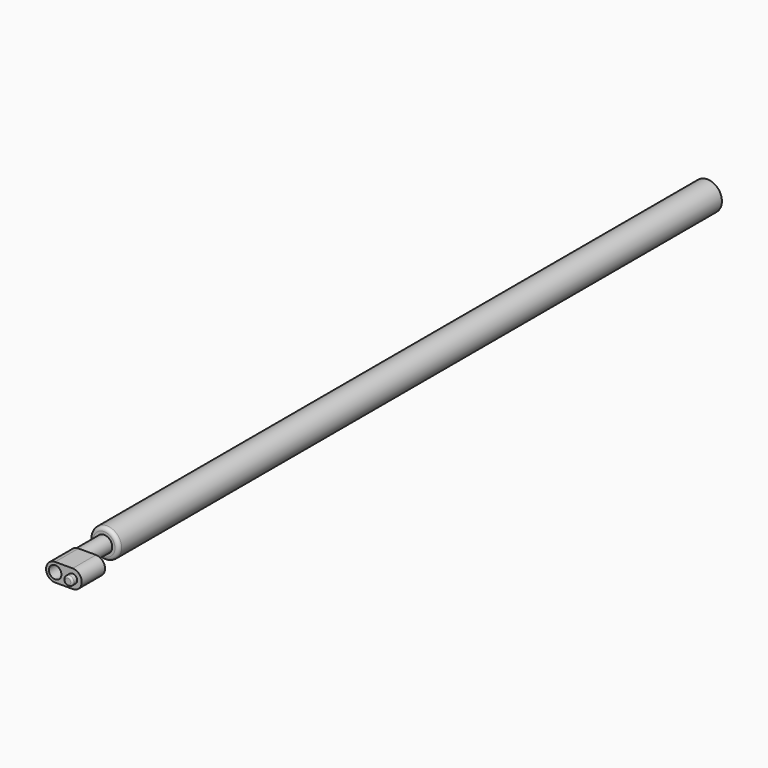
from build123d import *
from build123d import SkipClean  # not in build123d's __all__

# Parameters (mm, degrees)
F0_R     = 2.7305
F1_DEPTH = 12.7
F2_R     = 3.5052
F3_DEPTH = 6.35
F4_R     = 1.9812
F5_DEPTH = 7.62
F6_R     = 3.5052
F6_R_2   = 2.7305
F7_DEPTH = 25.4
F8_R     = 1.9812
F9_DEPTH = 10.16
F10_R    = 0.762


# Not quite as in the source:
# - after a boolean that leaves OpenCascade's solid faulty, fix() repairs it


with BuildPart() as f1:
    # F0 (on Front) → F1 (new body)
    with BuildSketch(Plane.XZ):
        with BuildLine():
            Line((7.62, 3.96875), (0, 3.96875))
            ThreePointArc((0, 3.96875), (-3.96875, 0), (0, -3.96875))
            Line((0, -3.96875), (7.62, -3.96875))
            ThreePointArc((7.62, -3.96875), (11.58875, 0), (7.62, 3.96875))
        make_face()
        Circle(F0_R, mode=Mode.SUBTRACT)
    extrude(amount=-F1_DEPTH)

    # F2 (on face) → F3 (cut)
    with BuildSketch(Plane(origin=(0, 12.7, 0), x_dir=(-1, 0, 0), z_dir=(0, 1, 0))):
        Circle(F2_R)
    extrude(amount=-F3_DEPTH, mode=Mode.SUBTRACT)

    # F4 (on face) → F5 (cut)
    with BuildSketch(Plane.XZ):
        with Locations((7.62, 0)):
            Circle(F4_R)
    extrude(amount=-F5_DEPTH, mode=Mode.SUBTRACT)

    # F6 (on face) → F7 (join)
    with BuildSketch(Plane(origin=(0, 6.35, 0), x_dir=(-1, 0, 0), z_dir=(0, 1, 0))):
        Circle(F6_R)
        Circle(F6_R_2, mode=Mode.SUBTRACT)
    with SkipClean():  # cleaning this boolean's faces spoils the solid; the shape is the same uncleaned
        extrude(amount=F7_DEPTH)

    # F8 (on face) → F9 (join)
    with BuildSketch(Plane.XZ.offset(-7.62)):
        with Locations((7.62, 0)):
            Circle(F8_R)
    extrude(amount=F9_DEPTH)

    add(f1.part.fix(), mode=Mode.REPLACE)

    # F10
    f10_edges = [f1.edges().sort_by_distance(p)[0] for p in [
        (5.6388, -2.54, 0),
    ]]
    fillet(f10_edges, radius=F10_R)

    # F11 (on Right) → F12 (revolve)
    with BuildSketch(Plane.YZ):
        with BuildLine():
            Line((26.67, 4.7625), (26.67, 3.556))
            Line((26.67, 3.556), (31.75, 3.556))
            Line((31.75, 3.556), (31.75, 2.7305))
            Line((31.75, 2.7305), (34.29, 2.7305))
            Line((34.29, 2.7305), (34.29, 4.7625))
            Line((34.29, 4.7625), (355.6, 4.7625))
            Line((355.6, 4.7625), (355.6, 6.35))
            Line((355.6, 6.35), (28.2575, 6.35))
            ThreePointArc((28.2575, 6.35), (27.1349679849, 5.8850320151), (26.67, 4.7625))
        make_face()
    revolve(axis=Axis((0, 6.35, 0), (0, -1, 0)))


solid = f1.part
